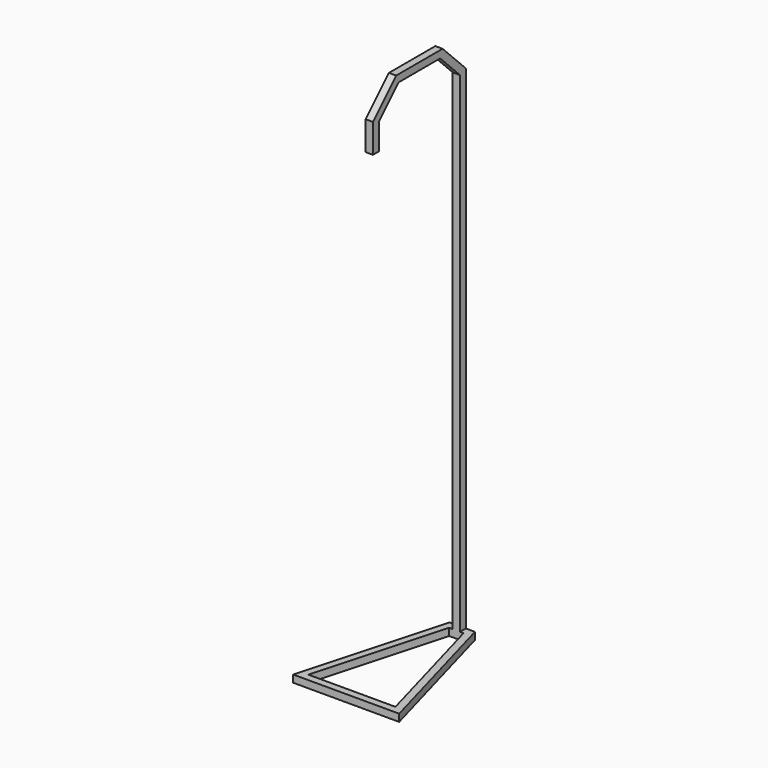
from build123d import *

# Parameters (mm, degrees)
F1_DEPTH = 25.4
F2_W     = 25.4
F2_H     = 25.4


with BuildPart() as f1:
    # F0 (on Top) → F1 (new body)
    with BuildSketch(Plane.XY):
        Polygon((44.7061754991, 508), (-44.7061754991, 508), (-185.8172866102, 0), (185.8172866102, 0), align=None)
        Polygon((-152.4, 25.4), (-25.4, 482.6), (25.4, 482.6), (152.4, 25.4), align=None, mode=Mode.SUBTRACT)
    extrude(amount=-F1_DEPTH)

    # F4: sweep along a path in F3
    with BuildLine(Plane.YZ) as f4_path:
        Line((508, 0), (508, 1727.2))
        Line((508, 1727.2), (406.4, 1828.8))
        Line((406.4, 1828.8), (203.2, 1828.8))
        Line((203.2, 1828.8), (101.6, 1727.2))
        Line((101.6, 1727.2), (101.6, 1625.6))
    # F2 (on Top) → F4 (sweep)
    with BuildSketch(Plane.XY):
        with Locations((0, 495.3)):
            Rectangle(F2_W, F2_H)
    sweep(path=f4_path.line, transition=Transition.RIGHT)


solid = f1.part
